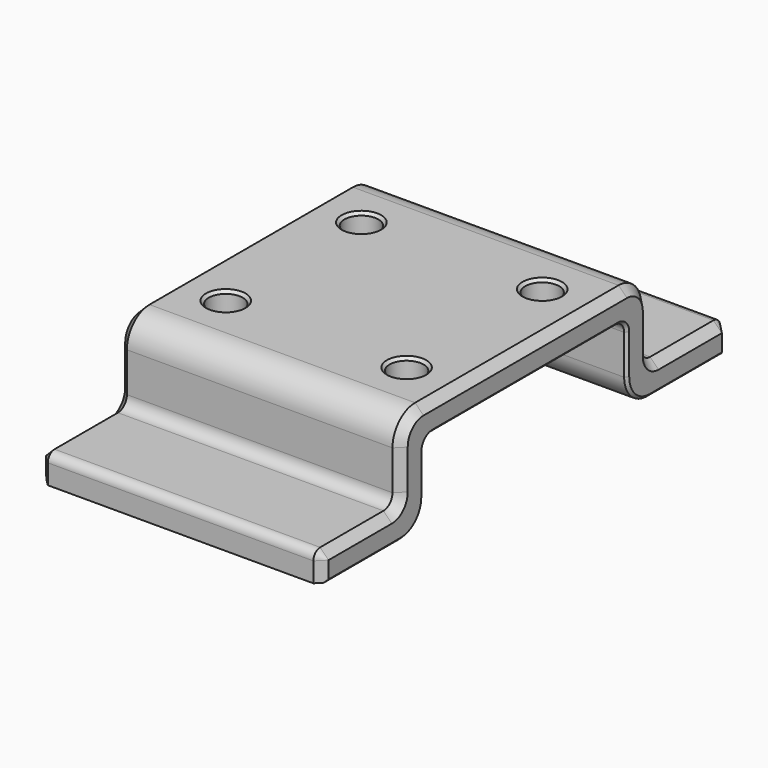
from build123d import *

# Parameters (mm, degrees)
F1_DEPTH = 100
F2_SIZE  = 2.99999
F3_SIZE  = 1
F4_R     = 6
F5_DEPTH = 10
F6_SIZE  = 1


# Not quite as in the source:
# - a fillet or chamfer is up to 0.001 mm smaller than in the source, because OpenCascade refuses the exact size


with BuildPart() as f1:
    # F0 (on Right) → F1 (new body)
    with BuildSketch(Plane.YZ):
        with BuildLine():
            Line((45, 36.1919924617), (0, 36.1919924617))
            Line((0, 36.1919924617), (0, 26.1919924617))
            Line((0, 26.1919924617), (41, 26.1919924617))
            ThreePointArc((41, 26.1919924617), (43.8284271247, 25.0204195864), (45, 22.1919924617))
            Line((45, 22.1919924617), (45, 8.2077106759))
            ThreePointArc((45, 8.2077106759), (47.9289321881, 1.136642864), (55, -1.7922893241))
            Line((55, -1.7922893241), (90, -1.7922893241))
            Line((90, -1.7922893241), (90, 5.2077106759))
            ThreePointArc((90, 5.2077106759), (89.1213203436, 7.3290310195), (87, 8.2077106759))
            Line((87, 8.2077106759), (59, 8.2077106759))
            ThreePointArc((59, 8.2077106759), (56.1715728753, 9.3792835511), (55, 12.2077106759))
            Line((55, 12.2077106759), (55, 26.1919924617))
            ThreePointArc((55, 26.1919924617), (52.0710678119, 33.2630602735), (45, 36.1919924617))
        make_face()
        with BuildLine():
            Line((0, 26.1919924617), (0, 36.1919924617))
            Line((0, 36.1919924617), (-45, 36.1919924617))
            ThreePointArc((-45, 36.1919924617), (-52.0710678119, 33.2630602735), (-55, 26.1919924617))
            Line((-55, 26.1919924617), (-55, 12.2077106759))
            ThreePointArc((-55, 12.2077106759), (-56.1715728753, 9.3792835511), (-59, 8.2077106759))
            Line((-59, 8.2077106759), (-87, 8.2077106759))
            ThreePointArc((-87, 8.2077106759), (-89.1213203436, 7.3290310195), (-90, 5.2077106759))
            Line((-90, 5.2077106759), (-90, -1.7922893241))
            Line((-90, -1.7922893241), (-55, -1.7922893241))
            ThreePointArc((-55, -1.7922893241), (-47.9289321881, 1.136642864), (-45, 8.2077106759))
            Line((-45, 8.2077106759), (-45, 22.1919924617))
            ThreePointArc((-45, 22.1919924617), (-43.8284271247, 25.0204195864), (-41, 26.1919924617))
            Line((-41, 26.1919924617), (0, 26.1919924617))
        make_face()
    extrude(amount=F1_DEPTH)

    # F2 (size 3 in the source; OpenCascade refuses exactly that, so slightly less here)
    f2_edges = [f1.edges().sort_by_distance(p)[0] for p in [
        (0, -90, 1.707711),
        (0, -89.12132, 7.329031),
        (0, -73, 8.207711),
        (0, -56.171573, 9.379284),
        (0, -55, 19.199852),
        (0, -52.071068, 33.26306),
        (0, 0, 36.191992),
        (0, 52.071068, 33.26306),
        (100, 0, 36.191992),
    ]]
    chamfer(f2_edges, length=F2_SIZE)

    # F3
    f3_edges = [f1.edges().sort_by_distance(p)[0] for p in [
        (100, 0, 26.191992),
        (0, 0, 26.191992),
    ]]
    chamfer(f3_edges, length=F3_SIZE)

    # F4 (on face) → F5 (cut)
    with BuildSketch(Plane.XY.offset(36.1919924617)):
        with Locations((18, -30)):
            Circle(F4_R)
        with Locations((82, -30)):
            Circle(F4_R)
        with Locations((82, 30)):
            Circle(F4_R)
        with Locations((18, 30)):
            Circle(F4_R)
    extrude(amount=-F5_DEPTH, mode=Mode.SUBTRACT)

    # F6
    f6_edges = [f1.edges().sort_by_distance(p)[0] for p in [
        (12, 30, 36.191992),
        (76, 30, 36.191992),
        (88, -30, 31.191992),
        (76, -30, 36.191992),
        (76, -30, 26.191992),
        (12, -30, 36.191992),
        (76, 30, 26.191992),
        (12, 30, 26.191992),
        (12, -30, 26.191992),
    ]]
    chamfer(f6_edges, length=F6_SIZE)


solid = f1.part
